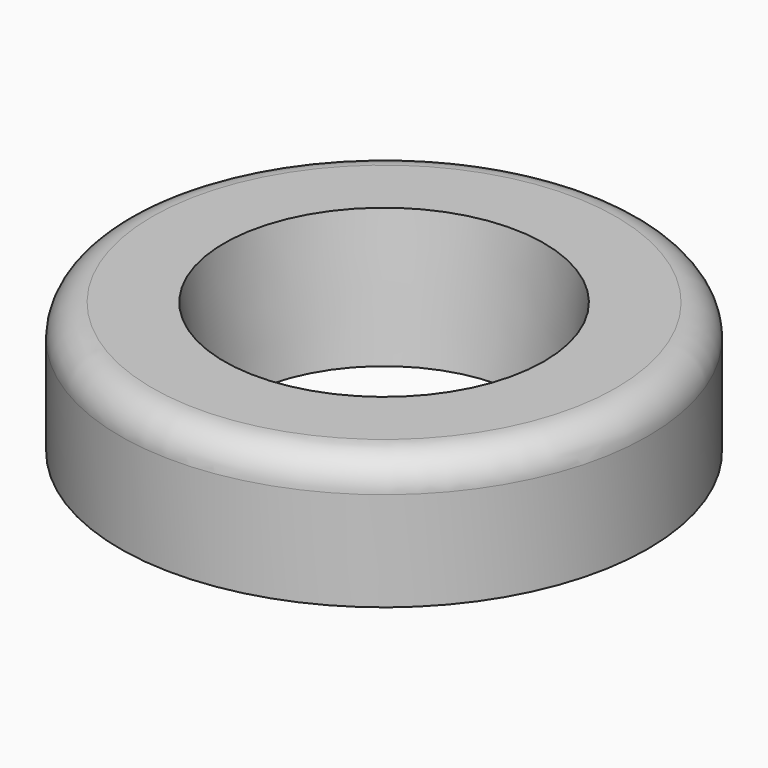
from build123d import *

# Parameters (mm, degrees)
F0_R     = 8.25
F0_R_2   = 4.5
F1_DEPTH = 4.1
F2_SIZE2 = 0.49999
F2_SIZE  = 4.09999
F3_R     = 1


# Not quite as in the source:
# - a fillet or chamfer is up to 0.001 mm smaller than in the source, because OpenCascade refuses the exact size


with BuildPart() as f1:
    # F0 (on Top) → F1 (new body)
    with BuildSketch(Plane.XY):
        Circle(F0_R)
        Circle(F0_R_2, mode=Mode.SUBTRACT)
    extrude(amount=F1_DEPTH)

    # F2 (size 4.1 and 0.5 in the source; OpenCascade refuses exactly that, so slightly less here)
    f2_edges = [f1.edges().sort_by_distance(p)[0] for p in [
        (-4.5, 0, 4.1),
    ]]
    f2_side = f1.faces().sort_by_distance((-4.5, 0, 2.05))[0]
    chamfer(f2_edges, length=F2_SIZE, length2=F2_SIZE2, reference=f2_side)

    # F3
    f3_edges = [f1.edges().sort_by_distance(p)[0] for p in [
        (-8.25, 0, 4.1),
    ]]
    fillet(f3_edges, radius=F3_R)


solid = f1.part
